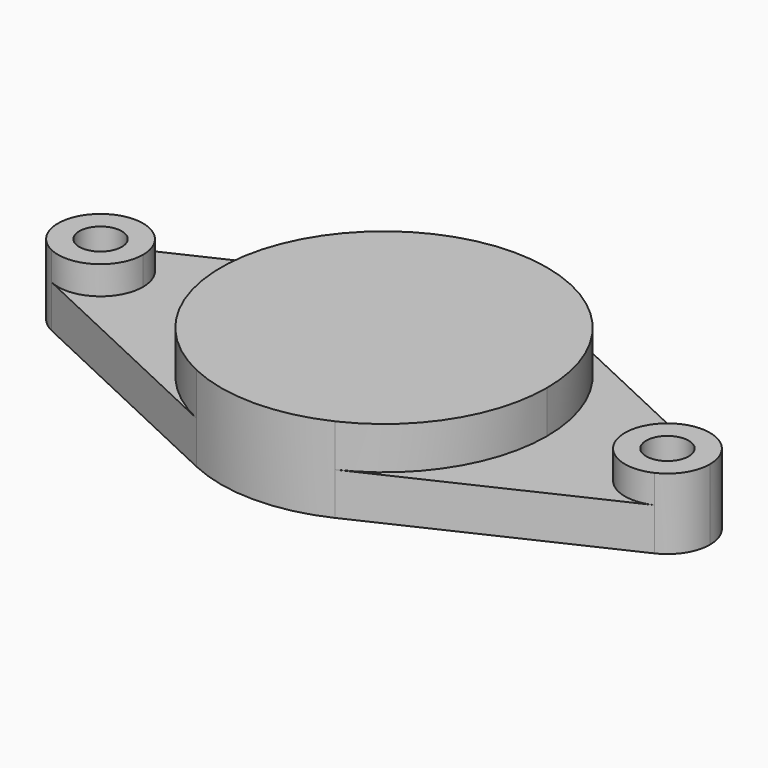
from build123d import *

# Parameters (mm, degrees)
F0_R     = 8.5
F1_DEPTH = 6
F2_DEPTH = 5
F0_R_2   = 1.5
F3_DEPTH = 5
F4_DEPTH = 3


with BuildPart() as f1:
    # F0 (on Top) → F1 (new body)
    with BuildSketch(Plane.XY):
        with BuildLine():
            ThreePointArc((4.8875, -10.4097235194), (9.7071172343, -6.1661880445), (11.5, 0))
            ThreePointArc((11.5, 0), (9.7071172343, 6.1661880445), (4.8875, 10.4097235194))
            ThreePointArc((4.8875, 10.4097235194), (0, 11.5), (-4.8875, 10.4097235194))
            ThreePointArc((-4.8875, 10.4097235194), (-11.5, 0), (-4.8875, -10.4097235194))
            ThreePointArc((-4.8875, -10.4097235194), (0, -11.5), (4.8875, -10.4097235194))
        make_face()
        Circle(F0_R, mode=Mode.SUBTRACT)
        Circle(F0_R)
    extrude(amount=F1_DEPTH)

    # F0 (on Top) → F2 (cut)
    with BuildSketch(Plane.XY):
        Circle(F0_R)
    extrude(amount=F2_DEPTH, mode=Mode.SUBTRACT)



with BuildPart() as f3:
    # F0 (on Top) → F3 (new body)
    with BuildSketch(Plane.XY):
        with BuildLine():
            ThreePointArc((-17, 0), (-18.3914292058, 2.5322914524), (-21.275, 2.7155800485))
            ThreePointArc((-21.275, 2.7155800485), (-23, 0), (-21.275, -2.7155800485))
            ThreePointArc((-21.275, -2.7155800485), (-18.3914292058, -2.5322914524), (-17, 0))
        make_face()
        with Locations((-20, 0)):
            Circle(F0_R_2, mode=Mode.SUBTRACT)
    extrude(amount=F3_DEPTH)


with BuildPart() as f3b:
    # F0 (on Top) → F3, piece 2 (new body)
    with BuildSketch(Plane.XY):
        with BuildLine():
            ThreePointArc((23, 0), (22.5322914524, 1.6085707942), (21.275, 2.7155800485))
            ThreePointArc((21.275, 2.7155800485), (17, 0), (21.275, -2.7155800485))
            ThreePointArc((21.275, -2.7155800485), (22.5322914524, -1.6085707942), (23, 0))
        make_face()
        with Locations((20, 0)):
            Circle(F0_R_2, mode=Mode.SUBTRACT)
    extrude(amount=F3_DEPTH)


with BuildPart() as f1_1:
    add(f1.part)

    add(f3.part)  # F4 merges F3

    add(f3b.part)  # F4 merges F3b
    # F0 (on Top) → F4 (join)
    with BuildSketch(Plane.XY):
        with BuildLine():
            ThreePointArc((-4.8875, -10.4097235194), (-11.5, 0), (-4.8875, 10.4097235194))
            Line((-4.8875, 10.4097235194), (-21.275, 2.7155800485))
            ThreePointArc((-21.275, 2.7155800485), (-18.3914292058, 2.5322914524), (-17, 0))
            ThreePointArc((-17, 0), (-18.3914292058, -2.5322914524), (-21.275, -2.7155800485))
            Line((-21.275, -2.7155800485), (-4.8875, -10.4097235194))
        make_face()
        with BuildLine():
            ThreePointArc((4.8875, 10.4097235194), (9.7071172343, 6.1661880445), (11.5, 0))
            ThreePointArc((11.5, 0), (9.7071172343, -6.1661880445), (4.8875, -10.4097235194))
            Line((4.8875, -10.4097235194), (21.275, -2.7155800485))
            ThreePointArc((21.275, -2.7155800485), (17, 0), (21.275, 2.7155800485))
            Line((21.275, 2.7155800485), (4.8875, 10.4097235194))
        make_face()
    extrude(amount=F4_DEPTH)


solid = f1_1.part
